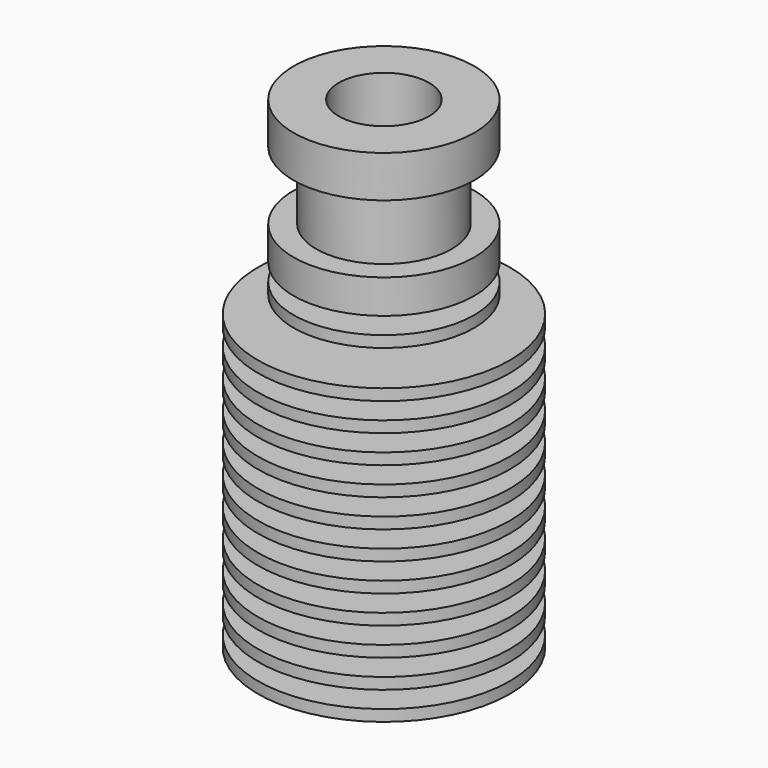
from build123d import *

# Parameters (mm, degrees)
F0_R         = 8
F1_DEPTH     = 3.7
F2_R         = 6
F3_DEPTH     = 6
F4_R         = 8
F5_DEPTH     = 3
F6_W         = 4
F6_H         = 1.5
F8_R         = 2.1
F9_DEPTH     = 42.7
F10_R        = 4
F11_DEPTH    = 6
F12_S5_R     = 4
F12_T6_DEPTH = 7
F13_R        = 3
F14_DEPTH    = 14.8
F15_S5_R     = 3
F15_T6_DEPTH = 6


# Not quite as in the source:
# - a fillet or chamfer that OpenCascade refuses, or shapes differently, is made with other operations: its cross-section is extruded or revolved along the edge and cut away or added


with BuildPart() as f1:
    # F0 (on Top) → F1 (new body)
    with BuildSketch(Plane.XY):
        Circle(F0_R)
    extrude(amount=-F1_DEPTH)

    # F2 (on face) → F3 (join)
    with BuildSketch(Plane(origin=(0, 0, -3.7), x_dir=(1, 0, 0), z_dir=(0, 0, -1))):
        Circle(F2_R)
    extrude(amount=F3_DEPTH)

    # F4 (on face) → F5 (join)
    with BuildSketch(Plane(origin=(0, 0, -9.7), x_dir=(1, 0, 0), z_dir=(0, 0, -1))):
        Circle(F4_R)
    extrude(amount=F5_DEPTH)

    # F6 (on Front) → F7 (revolve)
    with BuildSketch(Plane.XZ):
        with Locations((2, -13.45)):
            Rectangle(F6_W, F6_H)
        Polygon((4, -14.2), (0, -14.2), (0, -15.2), (4.0727272727, -15.2), (8, -15.2), (8, -14.2), align=None)
        Polygon((4.0727272727, -15.2), (0, -15.2), (0, -16.7), (4.1818181818, -16.7), align=None)
        Polygon((4.1818181818, -16.7), (0, -16.7), (0, -17.7), (4.2545454545, -17.7), (11.15, -17.7), (11.15, -16.7), align=None)
        Polygon((4.2545454545, -17.7), (0, -17.7), (0, -19.2), (4.3636363636, -19.2), align=None)
        Polygon((4.3636363636, -19.2), (0, -19.2), (0, -20.2), (4.4363636364, -20.2), (11.15, -20.2), (11.15, -19.2), align=None)
        Polygon((4.4363636364, -20.2), (0, -20.2), (0, -21.7), (4.5454545455, -21.7), align=None)
        Polygon((4.5454545455, -21.7), (0, -21.7), (0, -22.7), (4.6181818182, -22.7), (11.15, -22.7), (11.15, -21.7), align=None)
        Polygon((4.6181818182, -22.7), (0, -22.7), (0, -24.2), (4.7272727273, -24.2), align=None)
        Polygon((4.7272727273, -24.2), (0, -24.2), (0, -25.2), (4.8, -25.2), (11.15, -25.2), (11.15, -24.2), align=None)
        Polygon((4.8, -25.2), (0, -25.2), (0, -26.7), (4.9090909091, -26.7), align=None)
        Polygon((4.9090909091, -26.7), (0, -26.7), (0, -27.7), (4.9818181818, -27.7), (11.15, -27.7), (11.15, -26.7), align=None)
        Polygon((4.9818181818, -27.7), (0, -27.7), (0, -29.2), (5.0909090909, -29.2), align=None)
        Polygon((5.0909090909, -29.2), (0, -29.2), (0, -30.2), (5.1636363636, -30.2), (11.15, -30.2), (11.15, -29.2), align=None)
        Polygon((5.1636363636, -30.2), (0, -30.2), (0, -31.7), (5.2727272727, -31.7), align=None)
        Polygon((5.2727272727, -31.7), (0, -31.7), (0, -32.7), (5.3454545455, -32.7), (11.15, -32.7), (11.15, -31.7), align=None)
        Polygon((5.3454545455, -32.7), (0, -32.7), (0, -34.2), (5.4545454545, -34.2), align=None)
        Polygon((5.4545454545, -34.2), (0, -34.2), (0, -35.2), (5.5272727273, -35.2), (11.15, -35.2), (11.15, -34.2), align=None)
        Polygon((5.5272727273, -35.2), (0, -35.2), (0, -36.7), (5.6363636364, -36.7), align=None)
        Polygon((5.6363636364, -36.7), (0, -36.7), (0, -37.7), (5.7090909091, -37.7), (11.15, -37.7), (11.15, -36.7), align=None)
        Polygon((5.7090909091, -37.7), (0, -37.7), (0, -39.2), (5.8181818182, -39.2), align=None)
        Polygon((5.8181818182, -39.2), (0, -39.2), (0, -40.2), (5.8909090909, -40.2), (11.15, -40.2), (11.15, -39.2), align=None)
        Polygon((5.8909090909, -40.2), (0, -40.2), (0, -41.7), (6, -41.7), align=None)
        Polygon((6, -41.7), (0, -41.7), (0, -42.7), (11.15, -42.7), (11.15, -41.7), align=None)
    revolve(axis=Axis((0, 0, -6.35), (0, 0, -1)))

    # F8 (on face) → F9 (cut)
    with BuildSketch(Plane.XY):
        Circle(F8_R)
    extrude(amount=-F9_DEPTH, mode=Mode.SUBTRACT)

    # F10 (on face) → F11 (cut)
    with BuildSketch(Plane.XY):
        Circle(F10_R)
    extrude(amount=-F11_DEPTH, mode=Mode.SUBTRACT)

    # F12: chamfer of 2 on 1 edges, made by hand


with BuildPart() as f12_tool2:
    # F12_s3 → F12_t4 (revolve)
    with BuildSketch(Plane.XZ):
        Polygon((4.1, -6), (2.1, -8), (2.1, -6), align=None)
    revolve(axis=Axis((0, 0, -6), (0, 0, 1)))

    # F12_s5 → F12_t6 (intersect, symmetric)
    with BuildSketch(Plane.XY.offset(-7)):
        Circle(F12_S5_R)
    extrude(amount=F12_T6_DEPTH, both=True, mode=Mode.INTERSECT)


with BuildPart() as f1_1:
    add(f1.part)

    # F12_t1: cut F12_tool2
    add(f12_tool2.part, mode=Mode.SUBTRACT)

    # F13 (on face) → F14 (cut)
    with BuildSketch(Plane(origin=(0, 0, -42.7), x_dir=(1, 0, 0), z_dir=(0, 0, -1))):
        Circle(F13_R)
    extrude(amount=-F14_DEPTH, mode=Mode.SUBTRACT)

    # F15: chamfer of 1 on 1 edges, made by hand


with BuildPart() as f15_tool2:
    # F15_s3 → F15_t4 (revolve)
    with BuildSketch(Plane.XZ):
        Polygon((2.1, -26.9), (3.1, -27.9), (2.1, -27.9), align=None)
    revolve(axis=Axis((0, 0, -27.9), (0, 0, 1)))

    # F15_s5 → F15_t6 (intersect, symmetric)
    with BuildSketch(Plane.XY.offset(-27.4)):
        Circle(F15_S5_R)
    extrude(amount=F15_T6_DEPTH, both=True, mode=Mode.INTERSECT)


with BuildPart() as f1_2:
    add(f1_1.part)

    # F15_t1: cut F15_tool2
    add(f15_tool2.part, mode=Mode.SUBTRACT)


solid = f1_2.part
